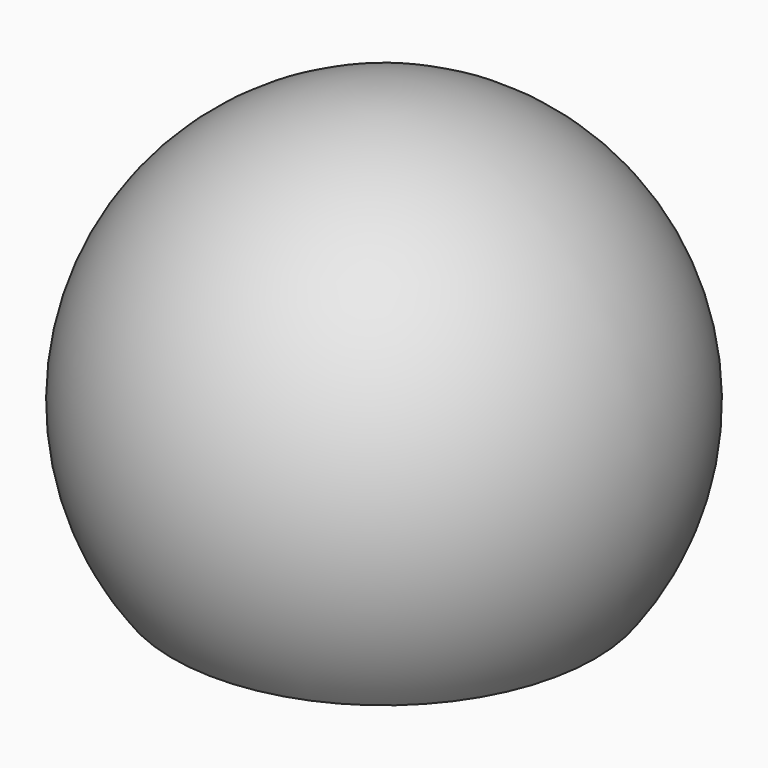
from build123d import *

# Parameters (mm, degrees)
F2_R      = 3.96875
F3_DEPTH  = 19.05
F3_FACE_R = 3.96875
F5_R      = 3.96875
F6_DEPTH  = 9.525
F7_R      = 3.96875
F8_DEPTH  = 3.175
F8_TAPER  = 60


# Not quite as in the source:
# - an extrude whose draft closes it to a point is written as a loft to that point


with BuildPart() as f1:
    # F0 (on Front) → F1 (revolve)
    with BuildSketch(Plane.XZ):
        with BuildLine():
            Line((0, 0), (12.7, 0))
            ThreePointArc((12.7, 0), (14.1990316571, 16.6245158286), (0, 25.4))
            Line((0, 25.4), (0, 0))
        make_face()
    revolve(axis=Axis((0, 0, 12.7), (0, 0, 1)))

    # F2 (on face) → F3 (cut)
    with BuildSketch(Plane(origin=(0, 0, 0), x_dir=(1, 0, 0), z_dir=(0, 0, -1))):
        Circle(F2_R)
    extrude(amount=-F3_DEPTH, mode=Mode.SUBTRACT)

    # F3_face (on face) → F4 section 0
    with BuildSketch(Plane(origin=(0, 0, 19.05), x_dir=(1, 0, 0), z_dir=(0, 0, -1)), mode=Mode.PRIVATE) as f4_s0:
        Circle(F3_FACE_R)
    loft([f4_s0.sketch, Vertex(0, 0, 23.01875)], ruled=True, mode=Mode.SUBTRACT)

    # F5 (on face) → F6 (cut)
    with BuildSketch(Plane(origin=(0, 0, 0), x_dir=(1, 0, 0), z_dir=(0, 0, -1))):
        Polygon((-8.5, 4.9074772881), (-8.5, -4.9074772881), (0, -9.8149545762), (8.5, -4.9074772881), (8.5, 4.9074772881), (0, 9.8149545762), align=None)
        Circle(F5_R, mode=Mode.SUBTRACT)
    extrude(amount=-F6_DEPTH, mode=Mode.SUBTRACT)

    # F7 (on face) → F8 (cut)
    with BuildSketch(Plane(origin=(0, 0, 9.525), x_dir=(1, 0, 0), z_dir=(0, 0, -1))):
        Polygon((8.5, 4.9074772881), (0, 9.8149545762), (-8.5, 4.9074772881), (-8.5, -4.9074772881), (0, -9.8149545762), (8.5, -4.9074772881), align=None)
        Circle(F7_R, mode=Mode.SUBTRACT)
        Circle(F7_R)
    extrude(amount=-F8_DEPTH, taper=F8_TAPER, mode=Mode.SUBTRACT)


solid = f1.part
